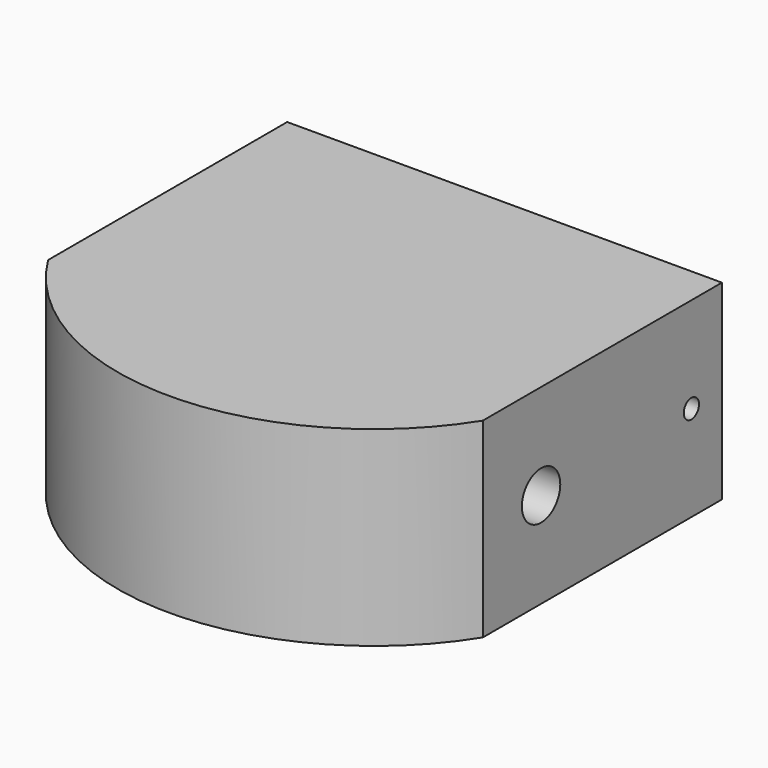
from build123d import *

# Parameters (mm, degrees)
F0_W         = 113.8667227506
F0_H         = 78.2720185816
F1_DEPTH     = 50
F2_R         = 6.2867981118
F2_R_2       = 2.5
F3_DEPTH     = 113.8677227506
F4_TEXT_SIZE = 22.4703907445
F5_DEPTH     = 12.5


# Not quite as in the source:
# - Text() gives the source's letters only with a copy of the font that has no kerning and outlines rounded to 1/6400 em; it was checked with that copy


with BuildPart() as f1:
    # F0 (on Top) → F1 (new body)
    with BuildSketch(Plane.XY):
        with BuildLine():
            ThreePointArc((-57.2852467089, -32.4923731387), (-0.3518853337, -64.0511000937), (56.5814760416, -32.4923731387))
            Line((56.5814760416, -32.4923731387), (-57.2852467089, -32.4923731387))
        make_face()
        with Locations((-0.3518853337, 6.6436361521)):
            Rectangle(F0_W, F0_H)
    extrude(amount=F1_DEPTH)

    # F2 (on face) → F3 (cut, through all)
    with BuildSketch(Plane.YZ.offset(56.5814760416)):
        with Locations((-13.428805396, 25)):
            Circle(F2_R)
        with Locations((35.779645443, 25)):
            Circle(F2_R_2)
    extrude(amount=-F3_DEPTH, mode=Mode.SUBTRACT)

    # F4 (on face) → F5 (cut, symmetric)
    with BuildSketch(Plane(origin=(0, 0, 0), x_dir=(1, 0, 0), z_dir=(0, 0, -1))):
        with Locations((-30.8704547845, -8.2562526759)):
            Text('D.A.D', F4_TEXT_SIZE, font='Open Sans', font_style=FontStyle.BOLD, text_align=(TextAlign.LEFT, TextAlign.BOTTOM))
    extrude(amount=F5_DEPTH, both=True, mode=Mode.SUBTRACT)


solid = f1.part
